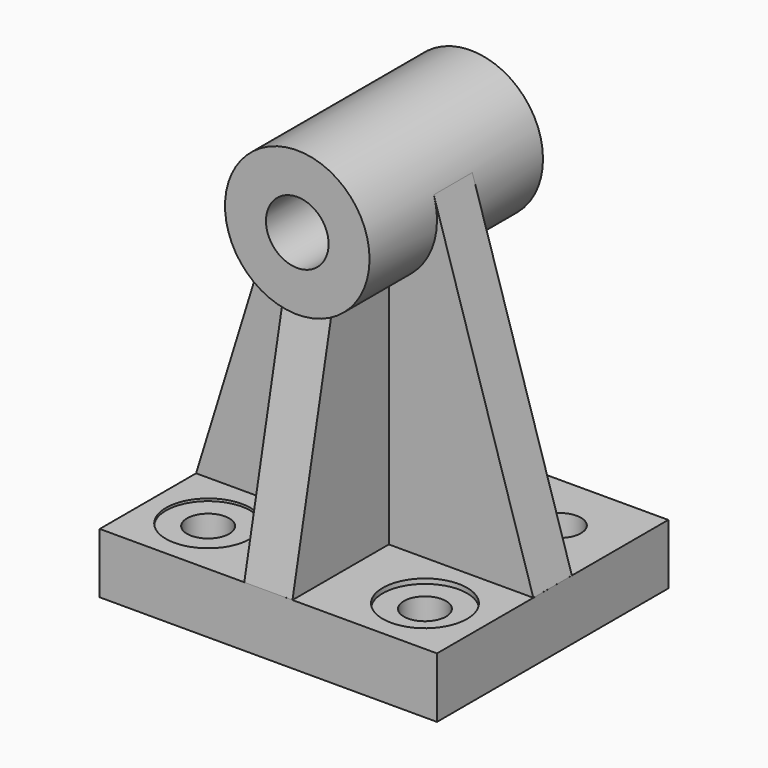
from build123d import *

# Parameters (mm, degrees)
F1_DEPTH  = 10
F3_DEPTH  = 60
F4_R      = 30
F4_R_2    = 13
F5_DEPTH  = 45
F7_DEPTH  = 10
F8_DEPTH  = 10
F9_DEPTH  = 5
F10_DEPTH = 5
F11_R     = 8.75
F12_DEPTH = 50
F13_R     = 17.5
F14_DEPTH = 1
F15_R     = 17.5
F16_DEPTH = 2


# Not quite as in the source:
# - a pattern or mirror of a feature is missing from the dataset's text; its kind, count and spacing are read off the source's solid


with BuildPart() as f1:
    # F0 (on Front) → F1 (new body, symmetric)
    with BuildSketch(Plane.XZ):
        with BuildLine():
            Line((-28.6642979162, 158.8520068331), (-70, 25))
            Line((-70, 25), (70, 25))
            Line((70, 25), (28.6642979162, 158.8520068331))
            ThreePointArc((28.6642979162, 158.8520068331), (29.6641950631, 154.4761067075), (30, 150))
            ThreePointArc((30, 150), (-4.4761067075, 120.3358049369), (-28.6642979162, 158.8520068331))
        make_face()
    extrude(amount=F1_DEPTH, both=True)

    # F2 (on Front) → F3 (join, symmetric)
    with BuildSketch(Plane.XZ):
        Polygon((70, 0), (70, 25.0431130097), (-70, 25), (-70, 0), align=None)
    extrude(amount=F3_DEPTH, both=True)

    # F4 (on Front) → F5 (join, symmetric)
    with BuildSketch(Plane.XZ):
        with Locations((0, 150)):
            Circle(F4_R)
        with Locations((0, 150)):
            Circle(F4_R_2, mode=Mode.SUBTRACT)
    extrude(amount=F5_DEPTH, both=True)

    # F6 (on Right) → F7 (join, symmetric)
    with BuildSketch(Plane.YZ):
        Polygon((60, 25), (40, 120), (10, 120), (10, 25), align=None)
    extrude(amount=F7_DEPTH, both=True)

    # F6 (on Right) → F8, piece 2 (join, symmetric)
    with BuildSketch(Plane.YZ):
        Polygon((-40, 120), (-60, 25), (-10.027478449, 25), (-10.027478449, 120), align=None)
    extrude(amount=F8_DEPTH, both=True)

    # F9 (add): a face of the model
    f9_faces = [f1.faces().sort_by_distance(p)[0] for p in [
        (5, 25, 120),
    ]]


with BuildPart() as f8:
    # F6 (on Right) → F8 (new body, symmetric)
    with BuildSketch(Plane.YZ):
        Polygon((60, 25), (40, 120), (10, 120), (10, 25), align=None)
    extrude(amount=F8_DEPTH, both=True)


with BuildPart() as f1_1:
    add(f1.part)

    add(f8.part)  # F9 merges F8
    f9 = extrude(f9_faces, amount=F9_DEPTH)

    # F9_copies: F9 across plane
    add(f9.mirror(Plane(origin=(0, 0, 0), x_dir=(0, 0, -1), z_dir=(-1, 0, 0))))

    # F10 (add): a face of the model
    f10_faces = [f1_1.faces().sort_by_distance(p)[0] for p in [
        (5, -25.0137392245, 120),
    ]]
    f10 = extrude(f10_faces, amount=F10_DEPTH)

    # F10_copies: F10 across plane
    add(f10.mirror(Plane(origin=(0, 0, 0), x_dir=(0, 0, -1), z_dir=(-1, 0, 0))))

    # F11 (on face) → F12 (cut)
    with BuildSketch(Plane(origin=(0, 0, 0), x_dir=(1, 0, 0), z_dir=(0, 0, -1))):
        with Locations((-45, -35)):
            Circle(F11_R)
        with Locations((-45, 35)):
            Circle(F11_R)
        with Locations((45, -35)):
            Circle(F11_R)
        with Locations((45, 35)):
            Circle(F11_R)
    extrude(amount=-F12_DEPTH, mode=Mode.SUBTRACT)

    # F13 (on face) → F14 (cut)
    with BuildSketch(Plane(origin=(-0.0077053893, 0, 25.021554132), x_dir=(0.9999999526, 0, 0.0003079501), z_dir=(-0.0003079501, 0, 0.9999999526))):
        with Locations((-44.992296744, -35)):
            Circle(F13_R)
        with BuildLine():
            add(Edge.make_bspline(
                [(-36.2422963292, -35), (-36.2422963292, -19.8445554338), (-49.3672969515, -27.4222777169), (-62.4922975738, -35), (-49.3672969515, -42.5777222831), (-36.2422963292, -50.1554445662), (-36.2422963292, -35)],
                knots=[3.1415926536, 3.1415926536, 3.1415926536, 5.235987756, 5.235987756, 7.3303828584, 7.3303828584, 9.4247779608, 9.4247779608, 9.4247779608], degree=2, weights=[1, 0.5, 1, 0.5, 1, 0.5, 1]))
        make_face(mode=Mode.SUBTRACT)
        with BuildLine():
            add(Edge.make_bspline(
                [(53.7577079383, -35), (53.7577079383, -19.8445554338), (40.632707316, -27.4222777169), (27.5077066937, -35), (40.632707316, -42.5777222831), (53.7577079383, -50.1554445662), (53.7577079383, -35)],
                knots=[3.1415926536, 3.1415926536, 3.1415926536, 5.235987756, 5.235987756, 7.3303828584, 7.3303828584, 9.4247779608, 9.4247779608, 9.4247779608], degree=2, weights=[1, 0.5, 1, 0.5, 1, 0.5, 1]))
        make_face()
        with BuildLine():
            add(Edge.make_bspline(
                [(-36.2422963292, -35), (-36.2422963292, -19.8445554338), (-49.3672969515, -27.4222777169), (-62.4922975738, -35), (-49.3672969515, -42.5777222831), (-36.2422963292, -50.1554445662), (-36.2422963292, -35)],
                knots=[3.1415926536, 3.1415926536, 3.1415926536, 5.235987756, 5.235987756, 7.3303828584, 7.3303828584, 9.4247779608, 9.4247779608, 9.4247779608], degree=2, weights=[1, 0.5, 1, 0.5, 1, 0.5, 1]))
        make_face()
    extrude(amount=-F14_DEPTH, mode=Mode.SUBTRACT)

    # F15 (on face) → F16 (cut)
    with BuildSketch(Plane(origin=(-0.0077053893, 0, 25.021554132), x_dir=(0.9999999526, 0, 0.0003079501), z_dir=(-0.0003079501, 0, 0.9999999526))):
        with Locations((45.0077075234, -35)):
            Circle(F15_R)
        with BuildLine():
            add(Edge.make_bspline(
                [(53.7577079383, -35), (53.7577079383, -19.8445554338), (40.632707316, -27.4222777169), (27.5077066937, -35), (40.632707316, -42.5777222831), (53.7577079383, -50.1554445662), (53.7577079383, -35)],
                knots=[3.1415926536, 3.1415926536, 3.1415926536, 5.235987756, 5.235987756, 7.3303828584, 7.3303828584, 9.4247779608, 9.4247779608, 9.4247779608], degree=2, weights=[1, 0.5, 1, 0.5, 1, 0.5, 1]))
        make_face(mode=Mode.SUBTRACT)
        with BuildLine():
            add(Edge.make_bspline(
                [(53.7577079383, -35), (53.7577079383, -19.8445554338), (40.632707316, -27.4222777169), (27.5077066937, -35), (40.632707316, -42.5777222831), (53.7577079383, -50.1554445662), (53.7577079383, -35)],
                knots=[3.1415926536, 3.1415926536, 3.1415926536, 5.235987756, 5.235987756, 7.3303828584, 7.3303828584, 9.4247779608, 9.4247779608, 9.4247779608], degree=2, weights=[1, 0.5, 1, 0.5, 1, 0.5, 1]))
        make_face()
    extrude(amount=-F16_DEPTH, mode=Mode.SUBTRACT)


solid = f1_1.part
